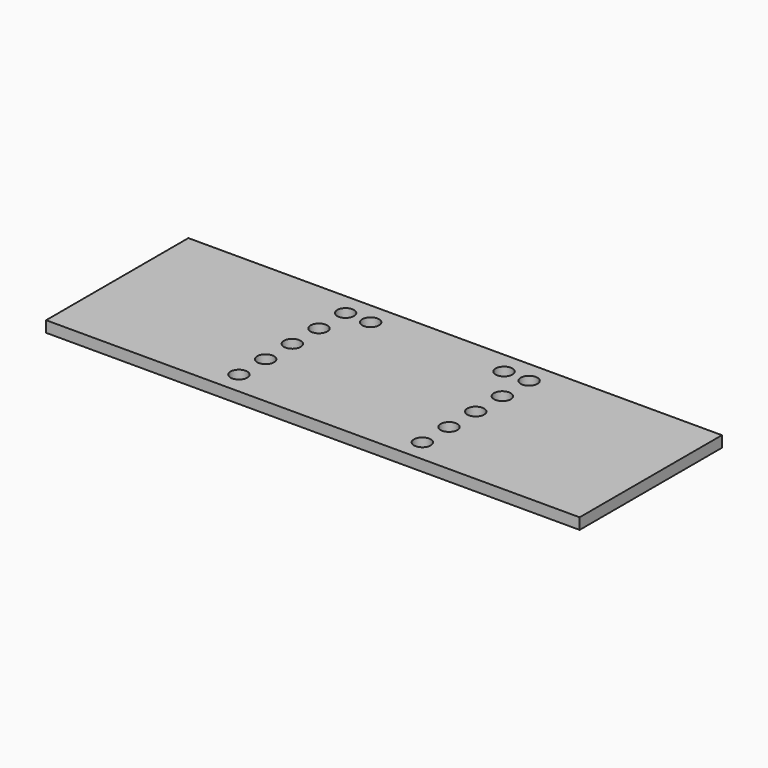
from build123d import *

# Parameters (mm, degrees)
F0_W     = 304.8
F0_H     = 101.6
F1_DEPTH = 6.35
F2_R     = 4.78155
F3_DEPTH = 6.35
F4_R     = 4.78155
F5_DEPTH = 6.351


# Not quite as in the source:
# - a feature names something its author has since deleted; it is built from what else it names


with BuildPart() as f1:
    # F0 (on Top) → F1 (new body)
    with BuildSketch(Plane.XY):
        Rectangle(F0_W, F0_H)
    extrude(amount=F1_DEPTH)

    # F2 (on face) → F3 (cut, through all)
    with BuildSketch(Plane.XY.offset(6.35)):
        with Locations((-52.3875, 38.1)):
            Circle(F2_R)
        with Locations((52.3875, 38.1)):
            Circle(F2_R)
        with Locations((-52.3875, 19.05)):
            Circle(F2_R)
        with Locations((52.3875, 19.05)):
            Circle(F2_R)
        with Locations((-52.3875, 0)):
            Circle(F2_R)
        with Locations((-52.3875, -19.05)):
            Circle(F2_R)
        with Locations((-52.3875, -38.1)):
            Circle(F2_R)
        with Locations((52.3875, 0)):
            Circle(F2_R)
        with Locations((52.3875, -19.05)):
            Circle(F2_R)
        with Locations((52.3875, -38.1)):
            Circle(F2_R)
    extrude(amount=-F3_DEPTH, mode=Mode.SUBTRACT)

    # F4 (on face) → F5 (cut, through all)
    with BuildSketch(Plane.XY.offset(6.35)):
        with Locations((-38.1, 38.1)):
            Circle(F4_R)
        with Locations((38.1, 38.1)):
            Circle(F4_R)
    extrude(amount=-F5_DEPTH, mode=Mode.SUBTRACT)


solid = f1.part
